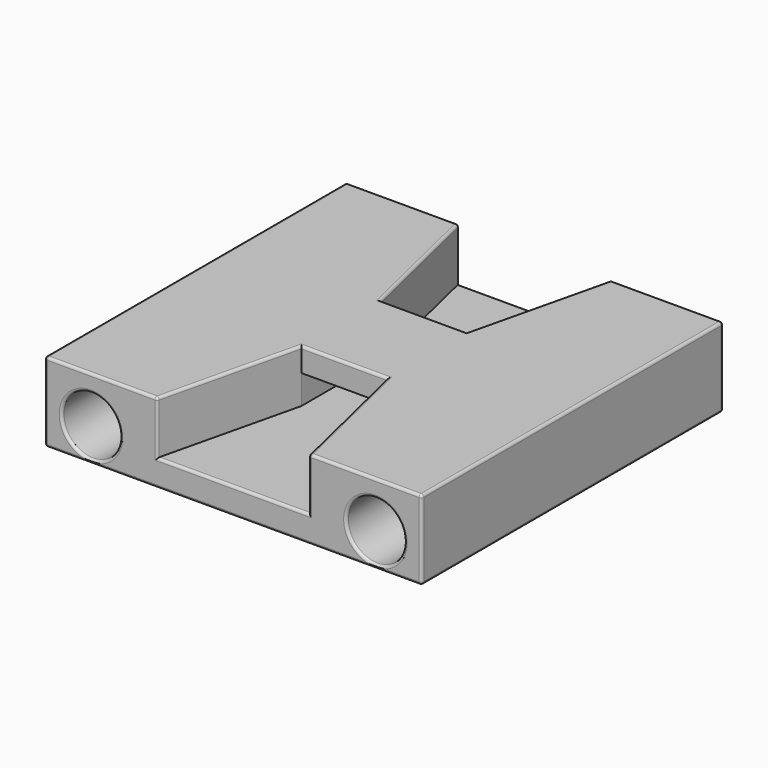
from build123d import *

# Parameters (mm, degrees)
F0_W          = 28.5
F0_H          = 28.5
F1_DEPTH      = 6
F2_W          = 6.5
F2_H          = 10.5
F3_DEPTH      = 4
F4_R          = 2.2
F5_DEPTH      = 28.501
F6_W          = 6.5
F6_H          = 2.2
F7_DEPTH      = 18.001
F8_T1_DEPTH   = 28.1
F8_T3_DEPTH   = 8.1410963279
F8_T5_DEPTH   = 8.1389034954
F8_T7_DEPTH   = 28.1
F8_T9_DEPTH   = 5.6
F8_T11_DEPTH  = 3.8
F8_S15_W      = 0.2
F8_S15_H      = 0.2
F8_T16_DEPTH  = 0.2
F8_S21_W      = 0.2
F8_S21_H      = 0.2
F8_T22_DEPTH  = 0.2
F8_T28_DEPTH  = 0.2
F8_T34_DEPTH  = 0.2
F8_S39_W      = 0.2
F8_S39_H      = 0.2
F8_T40_DEPTH  = 0.2
F8_S45_W      = 0.2
F8_S45_H      = 0.2
F8_T46_DEPTH  = 0.2
F8_T52_DEPTH  = 0.2
F8_T58_DEPTH  = 0.2
F8_S63_W      = 0.2
F8_S63_H      = 0.2
F8_T64_DEPTH  = 0.2
F8_S69_W      = 0.2
F8_S69_H      = 0.2
F8_T70_DEPTH  = 0.2
F8_S75_W      = 0.2
F8_S75_H      = 0.2
F8_T76_DEPTH  = 0.2
F8_S81_W      = 0.2
F8_S81_H      = 0.2
F8_T82_DEPTH  = 0.2
F8_T88_DEPTH  = 11.1357777684
F8_T93_DEPTH  = 7.5
F8_T99_DEPTH  = 11.13632618
F8_T104_DEPTH = 11.13632618
F8_T109_DEPTH = 7.5
F8_T115_DEPTH = 11.1357777684
F8_T120_DEPTH = 12.5041169338
F8_T130_DEPTH = 12.5041169338
F8_T141_DEPTH = 11.1357777684
F8_T145_DEPTH = 7.5
F8_T152_DEPTH = 7.5
F8_T156_DEPTH = 11.13632618
F8_T163_DEPTH = 7.5
F8_T167_DEPTH = 11.13632618
F8_T174_DEPTH = 7.5
F8_T178_DEPTH = 11.1357777684
F8_T185_DEPTH = 4.1948947572
F8_T189_DEPTH = 12.5041169338
F8_T196_DEPTH = 4.1948133503
F8_T200_DEPTH = 12.5041169338
F8_T207_DEPTH = 4.1948133503
F8_T211_DEPTH = 12.5041169338
F8_T218_DEPTH = 12.5041169338
F8_T222_DEPTH = 4.1948947572


# Not quite as in the source:
# - a fillet or chamfer that OpenCascade refuses, or shapes differently, is made with other operations: its cross-section is extruded or revolved along the edge and cut away or added


with BuildPart() as f1:
    # F0 (on Top) → F1 (new body)
    with BuildSketch(Plane.XY):
        Rectangle(F0_W, F0_H)
    extrude(amount=F1_DEPTH)

    # F2 (on face) → F3 (cut)
    with BuildSketch(Plane.XY.offset(6)):
        with Locations((0, 9)):
            Rectangle(F2_W, F2_H)
        Polygon((3.25, 14.25), (3.25, 3.75), (5.7531711645, 14.25), align=None)
        Polygon((-5.7509457693, 14.25), (-3.25, 3.75), (-3.25, 14.25), align=None)
        Polygon((-5.7509457693, -14.25), (-3.25, -14.25), (-3.25, -3.75), align=None)
        with Locations((0, -9)):
            Rectangle(F2_W, F2_H)
        Polygon((3.25, -3.75), (3.25, -14.25), (5.7531711645, -14.25), align=None)
    extrude(amount=-F3_DEPTH, mode=Mode.SUBTRACT)

    # F4 (on face) → F5 (cut, through all)
    with BuildSketch(Plane.XZ.offset(14.25)):
        with Locations((-10.75, 2.5)):
            Circle(F4_R)
        with Locations((10.75, 2.5)):
            Circle(F4_R)
    extrude(amount=-F5_DEPTH, mode=Mode.SUBTRACT)

    # F6 (on face) → F7 (cut, through all)
    with BuildSketch(Plane.XZ.offset(3.75)):
        with Locations((0, 3.1)):
            Rectangle(F6_W, F6_H)
    extrude(amount=-F7_DEPTH, mode=Mode.SUBTRACT)

    # F8: fillet of radius 0.2 on 30 edges, made by hand

    # F8_s2 → F8_t1 (cut)
    with BuildSketch(Plane.XZ.offset(-14.05)):
        with BuildLine():
            ThreePointArc((-14.05, 6), (-14.1914213562, 5.9414213562), (-14.25, 5.8))
            Line((-14.25, 5.8), (-14.25, 6))
            Line((-14.25, 6), (-14.05, 6))
        make_face()
        with BuildLine():
            ThreePointArc((14.05, 6), (14.1914213562, 5.9414213562), (14.25, 5.8))
            Line((14.25, 5.8), (14.25, 6))
            Line((14.25, 6), (14.05, 6))
        make_face()
        with BuildLine():
            ThreePointArc((14.25, 0.2), (14.1914213562, 0.0585786438), (14.05, 0))
            Line((14.05, 0), (14.25, 0))
            Line((14.25, 0), (14.25, 0.2))
        make_face()
        with BuildLine():
            ThreePointArc((-14.25, 0.2), (-14.1914213562, 0.0585786438), (-14.05, 0))
            Line((-14.05, 0), (-14.25, 0))
            Line((-14.25, 0), (-14.25, 0.2))
        make_face()
    extrude(amount=F8_T1_DEPTH, mode=Mode.SUBTRACT)

    # F8_s4 → F8_t3 (cut)
    with BuildSketch(Plane.YZ.offset(-14.05)):
        with BuildLine():
            ThreePointArc((14.25, 5.8), (14.1914213562, 5.9414213562), (14.05, 6))
            Line((14.05, 6), (14.25, 6))
            Line((14.25, 6), (14.25, 5.8))
        make_face()
        with BuildLine():
            ThreePointArc((-14.25, 5.8), (-14.1914213562, 5.9414213562), (-14.05, 6))
            Line((-14.05, 6), (-14.25, 6))
            Line((-14.25, 6), (-14.25, 5.8))
        make_face()
    extrude(amount=F8_T3_DEPTH, mode=Mode.SUBTRACT)

    # F8_s6 → F8_t5 (cut)
    with BuildSketch(Plane.YZ.offset(5.9110965046)):
        with BuildLine():
            ThreePointArc((14.25, 5.8), (14.1914213562, 5.9414213562), (14.05, 6))
            Line((14.05, 6), (14.25, 6))
            Line((14.25, 6), (14.25, 5.8))
        make_face()
        with BuildLine():
            ThreePointArc((-14.25, 5.8), (-14.1914213562, 5.9414213562), (-14.05, 6))
            Line((-14.05, 6), (-14.25, 6))
            Line((-14.25, 6), (-14.25, 5.8))
        make_face()
    extrude(amount=F8_T5_DEPTH, mode=Mode.SUBTRACT)

    # F8_s8 → F8_t7 (cut)
    with BuildSketch(Plane.YZ.offset(-14.05)):
        with BuildLine():
            ThreePointArc((-14.25, 0.2), (-14.1914213562, 0.0585786438), (-14.05, 0))
            Line((-14.05, 0), (-14.25, 0))
            Line((-14.25, 0), (-14.25, 0.2))
        make_face()
        with BuildLine():
            ThreePointArc((14.25, 0.2), (14.1914213562, 0.0585786438), (14.05, 0))
            Line((14.05, 0), (14.25, 0))
            Line((14.25, 0), (14.25, 0.2))
        make_face()
    extrude(amount=F8_T7_DEPTH, mode=Mode.SUBTRACT)

    # F8_s10 → F8_t9 (cut)
    with BuildSketch(Plane.XY.offset(0.2)):
        with BuildLine():
            ThreePointArc((-14.05, -14.25), (-14.1914213562, -14.1914213562), (-14.25, -14.05))
            Line((-14.25, -14.05), (-14.25, -14.25))
            Line((-14.25, -14.25), (-14.05, -14.25))
        make_face()
        with BuildLine():
            ThreePointArc((14.05, -14.25), (14.1914213562, -14.1914213562), (14.25, -14.05))
            Line((14.25, -14.05), (14.25, -14.25))
            Line((14.25, -14.25), (14.05, -14.25))
        make_face()
        with BuildLine():
            ThreePointArc((14.05, 14.25), (14.1914213562, 14.1914213562), (14.25, 14.05))
            Line((14.25, 14.05), (14.25, 14.25))
            Line((14.25, 14.25), (14.05, 14.25))
        make_face()
        with BuildLine():
            ThreePointArc((-14.05, 14.25), (-14.1914213562, 14.1914213562), (-14.25, 14.05))
            Line((-14.25, 14.05), (-14.25, 14.25))
            Line((-14.25, 14.25), (-14.05, 14.25))
        make_face()
    extrude(amount=F8_T9_DEPTH, mode=Mode.SUBTRACT)

    # F8_s12 → F8_t11 (cut)
    with BuildSketch(Plane.XY.offset(2)):
        with BuildLine():
            ThreePointArc((-5.9089036721, -14.25), (-5.7849442794, -14.2069524417), (-5.7143463785, -14.0963406896))
            Line((-5.7143463785, -14.0963406896), (-5.7509457693, -14.25))
            Line((-5.7509457693, -14.25), (-5.9089036721, -14.25))
        make_face()
        with BuildLine():
            ThreePointArc((5.9110965046, -14.25), (5.7871528513, -14.2069648712), (5.7165485088, -14.0963797079))
            Line((5.7165485088, -14.0963797079), (5.7531711645, -14.25))
            Line((5.7531711645, -14.25), (5.9110965046, -14.25))
        make_face()
        with BuildLine():
            ThreePointArc((5.9110965046, 14.25), (5.7871528513, 14.2069648712), (5.7165485088, 14.0963797079))
            Line((5.7165485088, 14.0963797079), (5.7531711645, 14.25))
            Line((5.7531711645, 14.25), (5.9110965046, 14.25))
        make_face()
        with BuildLine():
            ThreePointArc((-5.9089036721, 14.25), (-5.7849442794, 14.2069524417), (-5.7143463785, 14.0963406896))
            Line((-5.7143463785, 14.0963406896), (-5.7509457693, 14.25))
            Line((-5.7509457693, 14.25), (-5.9089036721, 14.25))
        make_face()
    extrude(amount=F8_T11_DEPTH, mode=Mode.SUBTRACT)


with BuildPart() as f8_tool14:
    # F8_s15 → F8_t16 (new body)
    with BuildSketch(Plane.YZ.offset(-14.05)):
        with Locations((14.15, 5.9)):
            Rectangle(F8_S15_W, F8_S15_H)
    extrude(amount=-F8_T16_DEPTH)

    # F8_s17 → F8_t18 (revolve, cut)
    with BuildSketch(Plane(origin=(-14.05, 14.05, 5.8), x_dir=(0, -0.7071067812, -0.7071067812), z_dir=(0, 0.7071067812, -0.7071067812))):
        with BuildLine():
            ThreePointArc((0, -0.2), (0.2, 0), (0, 0.2))
            Line((0, 0.2), (0, -0.2))
        make_face()
    revolve(axis=Axis((-14.05, 14.05, 5.8), (-1, 0, 0)), mode=Mode.SUBTRACT)


with BuildPart() as f1_1:
    add(f1.part)

    # F8_t13: cut F8_tool14
    add(f8_tool14.part, mode=Mode.SUBTRACT)


with BuildPart() as f8_tool20:
    # F8_s21 → F8_t22 (new body)
    with BuildSketch(Plane.YZ.offset(-14.05)):
        with Locations((-14.15, 5.9)):
            Rectangle(F8_S21_W, F8_S21_H)
    extrude(amount=-F8_T22_DEPTH)

    # F8_s23 → F8_t24 (revolve, cut)
    with BuildSketch(Plane(origin=(-14.05, -14.05, 5.8), x_dir=(0, 0.7071067812, -0.7071067812), z_dir=(0, 0.7071067812, 0.7071067812))):
        with BuildLine():
            ThreePointArc((0, -0.2), (0.2, 0), (0, 0.2))
            Line((0, 0.2), (0, -0.2))
        make_face()
    revolve(axis=Axis((-14.05, -14.05, 5.8), (-1, 0, 0)), mode=Mode.SUBTRACT)


with BuildPart() as f1_2:
    add(f1_1.part)

    # F8_t19: cut F8_tool20
    add(f8_tool20.part, mode=Mode.SUBTRACT)


with BuildPart() as f8_tool26:
    # F8_s27 → F8_t28 (new body)
    with BuildSketch(Plane.XY.offset(5.8)):
        Polygon((-5.9089036721, 14.05), (-5.9089036721, 14.25), (-5.7509457693, 14.25), (-5.7143463785, 14.0963406896), align=None)
    extrude(amount=F8_T28_DEPTH)

    # F8_s29 → F8_t30 (revolve, cut)
    with BuildSketch(Plane(origin=(-5.9089036721, 14.05, 5.8), x_dir=(-0.6197969636, -0.7847622085, 0), z_dir=(-0.7847622085, 0.6197969636, 0))):
        with BuildLine():
            ThreePointArc((0, -0.2), (0.2, 0), (0, 0.2))
            Line((0, 0.2), (0, -0.2))
        make_face()
    revolve(axis=Axis((-5.9089036721, 14.05, 5.8), (0, 0, 1)), mode=Mode.SUBTRACT)


with BuildPart() as f1_3:
    add(f1_2.part)

    # F8_t25: cut F8_tool26
    add(f8_tool26.part, mode=Mode.SUBTRACT)


with BuildPart() as f8_tool32:
    # F8_s33 → F8_t34 (new body)
    with BuildSketch(Plane.XY.offset(5.8)):
        Polygon((5.9110965046, 14.05), (5.7165485088, 14.0963797079), (5.7531711645, 14.25), (5.9110965046, 14.25), align=None)
    extrude(amount=F8_T34_DEPTH)

    # F8_s35 → F8_t36 (revolve, cut)
    with BuildSketch(Plane(origin=(5.9110965046, 14.05, 5.8), x_dir=(0.6197182668, -0.784824356, 0), z_dir=(-0.784824356, -0.6197182668, 0))):
        with BuildLine():
            ThreePointArc((0, -0.2), (0.2, 0), (0, 0.2))
            Line((0, 0.2), (0, -0.2))
        make_face()
    revolve(axis=Axis((5.9110965046, 14.05, 5.8), (0, 0, 1)), mode=Mode.SUBTRACT)


with BuildPart() as f1_4:
    add(f1_3.part)

    # F8_t31: cut F8_tool32
    add(f8_tool32.part, mode=Mode.SUBTRACT)


with BuildPart() as f8_tool38:
    # F8_s39 → F8_t40 (new body)
    with BuildSketch(Plane.XZ.offset(-14.05)):
        with Locations((14.15, 5.9)):
            Rectangle(F8_S39_W, F8_S39_H)
    extrude(amount=-F8_T40_DEPTH)

    # F8_s41 → F8_t42 (revolve, cut)
    with BuildSketch(Plane(origin=(14.05, 14.05, 5.8), x_dir=(-0.7071067812, 0, -0.7071067812), z_dir=(0.7071067812, 0, -0.7071067812))):
        with BuildLine():
            ThreePointArc((0, -0.2), (0.2, 0), (0, 0.2))
            Line((0, 0.2), (0, -0.2))
        make_face()
    revolve(axis=Axis((14.05, 14.05, 5.8), (0, 1, 0)), mode=Mode.SUBTRACT)


with BuildPart() as f1_5:
    add(f1_4.part)

    # F8_t37: cut F8_tool38
    add(f8_tool38.part, mode=Mode.SUBTRACT)


with BuildPart() as f8_tool44:
    # F8_s45 → F8_t46 (new body)
    with BuildSketch(Plane.XZ.offset(14.05)):
        with Locations((14.15, 5.9)):
            Rectangle(F8_S45_W, F8_S45_H)
    extrude(amount=F8_T46_DEPTH)

    # F8_s47 → F8_t48 (revolve, cut)
    with BuildSketch(Plane(origin=(14.05, -14.05, 5.8), x_dir=(-0.7071067812, 0, -0.7071067812), z_dir=(-0.7071067812, 0, 0.7071067812))):
        with BuildLine():
            ThreePointArc((0, -0.2), (0.2, 0), (0, 0.2))
            Line((0, 0.2), (0, -0.2))
        make_face()
    revolve(axis=Axis((14.05, -14.05, 5.8), (0, -1, 0)), mode=Mode.SUBTRACT)


with BuildPart() as f1_6:
    add(f1_5.part)

    # F8_t43: cut F8_tool44
    add(f8_tool44.part, mode=Mode.SUBTRACT)


with BuildPart() as f8_tool50:
    # F8_s51 → F8_t52 (new body)
    with BuildSketch(Plane.XY.offset(5.8)):
        Polygon((5.9110965046, -14.05), (5.9110965046, -14.25), (5.7531711645, -14.25), (5.7165485088, -14.0963797079), align=None)
    extrude(amount=F8_T52_DEPTH)

    # F8_s53 → F8_t54 (revolve, cut)
    with BuildSketch(Plane(origin=(5.9110965046, -14.05, 5.8), x_dir=(0.6197182668, 0.784824356, 0), z_dir=(0.784824356, -0.6197182668, 0))):
        with BuildLine():
            ThreePointArc((0, -0.2), (0.2, 0), (0, 0.2))
            Line((0, 0.2), (0, -0.2))
        make_face()
    revolve(axis=Axis((5.9110965046, -14.05, 5.8), (0, 0, 1)), mode=Mode.SUBTRACT)


with BuildPart() as f1_7:
    add(f1_6.part)

    # F8_t49: cut F8_tool50
    add(f8_tool50.part, mode=Mode.SUBTRACT)


with BuildPart() as f8_tool56:
    # F8_s57 → F8_t58 (new body)
    with BuildSketch(Plane.XY.offset(5.8)):
        Polygon((-5.9089036721, -14.05), (-5.9089036721, -14.25), (-5.7509457693, -14.25), (-5.7143463785, -14.0963406896), align=None)
    extrude(amount=F8_T58_DEPTH)

    # F8_s59 → F8_t60 (revolve, cut)
    with BuildSketch(Plane(origin=(-5.9089036721, -14.05, 5.8), x_dir=(-0.6197969636, 0.7847622085, 0), z_dir=(0.7847622085, 0.6197969636, 0))):
        with BuildLine():
            ThreePointArc((0, -0.2), (0.2, 0), (0, 0.2))
            Line((0, 0.2), (0, -0.2))
        make_face()
    revolve(axis=Axis((-5.9089036721, -14.05, 5.8), (0, 0, 1)), mode=Mode.SUBTRACT)


with BuildPart() as f1_8:
    add(f1_7.part)

    # F8_t55: cut F8_tool56
    add(f8_tool56.part, mode=Mode.SUBTRACT)


with BuildPart() as f8_tool62:
    # F8_s63 → F8_t64 (new body)
    with BuildSketch(Plane.XZ.offset(14.05)):
        with Locations((-14.15, 0.1)):
            Rectangle(F8_S63_W, F8_S63_H)
    extrude(amount=F8_T64_DEPTH)

    # F8_s65 → F8_t66 (revolve, cut)
    with BuildSketch(Plane(origin=(-14.05, -14.05, 0.2), x_dir=(0.7071067812, 0, 0.7071067812), z_dir=(0.7071067812, 0, -0.7071067812))):
        with BuildLine():
            ThreePointArc((0, -0.2), (0.2, 0), (0, 0.2))
            Line((0, 0.2), (0, -0.2))
        make_face()
    revolve(axis=Axis((-14.05, -14.05, 0.2), (0, -1, 0)), mode=Mode.SUBTRACT)


with BuildPart() as f1_9:
    add(f1_8.part)

    # F8_t61: cut F8_tool62
    add(f8_tool62.part, mode=Mode.SUBTRACT)


with BuildPart() as f8_tool68:
    # F8_s69 → F8_t70 (new body)
    with BuildSketch(Plane.XZ.offset(14.05)):
        with Locations((14.15, 0.1)):
            Rectangle(F8_S69_W, F8_S69_H)
    extrude(amount=F8_T70_DEPTH)

    # F8_s71 → F8_t72 (revolve, cut)
    with BuildSketch(Plane(origin=(14.05, -14.05, 0.2), x_dir=(-0.7071067812, 0, 0.7071067812), z_dir=(0.7071067812, 0, 0.7071067812))):
        with BuildLine():
            ThreePointArc((0, -0.2), (0.2, 0), (0, 0.2))
            Line((0, 0.2), (0, -0.2))
        make_face()
    revolve(axis=Axis((14.05, -14.05, 0.2), (0, -1, 0)), mode=Mode.SUBTRACT)


with BuildPart() as f1_10:
    add(f1_9.part)

    # F8_t67: cut F8_tool68
    add(f8_tool68.part, mode=Mode.SUBTRACT)


with BuildPart() as f8_tool74:
    # F8_s75 → F8_t76 (new body)
    with BuildSketch(Plane.XY.offset(0.2)):
        with Locations((14.15, 14.15)):
            Rectangle(F8_S75_W, F8_S75_H)
    extrude(amount=-F8_T76_DEPTH)

    # F8_s77 → F8_t78 (revolve, cut)
    with BuildSketch(Plane(origin=(14.05, 14.05, 0.2), x_dir=(-0.7071067812, -0.7071067812, 0), z_dir=(0.7071067812, -0.7071067812, 0))):
        with BuildLine():
            ThreePointArc((0, -0.2), (0.2, 0), (0, 0.2))
            Line((0, 0.2), (0, -0.2))
        make_face()
    revolve(axis=Axis((14.05, 14.05, 0.2), (0, 0, -1)), mode=Mode.SUBTRACT)


with BuildPart() as f1_11:
    add(f1_10.part)

    # F8_t73: cut F8_tool74
    add(f8_tool74.part, mode=Mode.SUBTRACT)


with BuildPart() as f8_tool80:
    # F8_s81 → F8_t82 (new body)
    with BuildSketch(Plane.YZ.offset(-14.05)):
        with Locations((14.15, 0.1)):
            Rectangle(F8_S81_W, F8_S81_H)
    extrude(amount=-F8_T82_DEPTH)

    # F8_s83 → F8_t84 (revolve, cut)
    with BuildSketch(Plane(origin=(-14.05, 14.05, 0.2), x_dir=(0, -0.7071067812, 0.7071067812), z_dir=(0, -0.7071067812, -0.7071067812))):
        with BuildLine():
            ThreePointArc((0, -0.2), (0.2, 0), (0, 0.2))
            Line((0, 0.2), (0, -0.2))
        make_face()
    revolve(axis=Axis((-14.05, 14.05, 0.2), (-1, 0, 0)), mode=Mode.SUBTRACT)


with BuildPart() as f1_12:
    add(f1_11.part)

    # F8_t79: cut F8_tool80
    add(f8_tool80.part, mode=Mode.SUBTRACT)


with BuildPart() as f8_tool86:
    # F8_s87 → F8_t88 (new body)
    with BuildSketch(Plane(origin=(-3.4840698832, 14.627559791, 0), x_dir=(0, 0, 1), z_dir=(0.2317034478, -0.972786468, 0))):
        with BuildLine():
            ThreePointArc((5.8, 2.2926680918), (5.9414213562, 2.3512467356), (6, 2.4926680918))
            Line((6, 2.4926680918), (6, 2.2926680918))
            Line((6, 2.2926680918), (5.8, 2.2926680918))
        make_face()
    extrude(amount=F8_T88_DEPTH)

    split(bisect_by=Plane.XZ.offset(-3.75), keep=Keep.BOTTOM)


with BuildPart() as f1_13:
    add(f1_12.part)

    # F8_t85: cut F8_tool86
    add(f8_tool86.part, mode=Mode.SUBTRACT)


with BuildPart() as f8_tool91:
    # F8_s92 → F8_t93 (new body)
    with BuildSketch(Plane.YZ.offset(-3.75)):
        with BuildLine():
            ThreePointArc((3.75, 5.8), (3.6914213562, 5.9414213562), (3.55, 6))
            Line((3.55, 6), (3.75, 6))
            Line((3.75, 6), (3.75, 5.8))
        make_face()
    extrude(amount=F8_T93_DEPTH)

    split(bisect_by=Plane(origin=(-2.2302764953, -0.5312191015, 0), x_dir=(0, 0, 1), z_dir=(0.972786468, 0.2317034478, 0)), keep=Keep.TOP)

    split(bisect_by=Plane(origin=(2.2293112911, -0.5314616896, 0), x_dir=(0, 0, 1), z_dir=(-0.9727399793, 0.2318985397, 0)), keep=Keep.TOP)


with BuildPart() as f1_14:
    add(f1_13.part)

    # F8_t90: cut F8_tool91
    add(f8_tool91.part, mode=Mode.SUBTRACT)


with BuildPart() as f8_tool97:
    # F8_s98 → F8_t99 (new body)
    with BuildSketch(Plane(origin=(0.9047394391, 3.7950916999, 0), x_dir=(0, 0, 1), z_dir=(0.2318985397, 0.9727399793, 0))):
        with BuildLine():
            ThreePointArc((5.8, 2.2917854088), (5.9414213562, 2.3503640526), (6, 2.4917854088))
            Line((6, 2.4917854088), (6, 2.2917854088))
            Line((6, 2.2917854088), (5.8, 2.2917854088))
        make_face()
    extrude(amount=F8_T99_DEPTH)

    split(bisect_by=Plane.XZ.offset(-3.75), keep=Keep.BOTTOM)


with BuildPart() as f1_15:
    add(f1_14.part)

    # F8_t96: cut F8_tool97
    add(f8_tool97.part, mode=Mode.SUBTRACT)


with BuildPart() as f8_tool102:
    # F8_s103 → F8_t104 (new body)
    with BuildSketch(Plane(origin=(3.4872372177, -14.6278413975, 0), x_dir=(0, 0, 1), z_dir=(-0.2318985397, 0.9727399793, 0))):
        with BuildLine():
            ThreePointArc((5.8, 2.2917854088), (5.9414213562, 2.3503640526), (6, 2.4917854088))
            Line((6, 2.4917854088), (6, 2.2917854088))
            Line((6, 2.2917854088), (5.8, 2.2917854088))
        make_face()
    extrude(amount=F8_T104_DEPTH)

    split(bisect_by=Plane.XZ.offset(3.75), keep=Keep.TOP)


with BuildPart() as f1_16:
    add(f1_15.part)

    # F8_t101: cut F8_tool102
    add(f8_tool102.part, mode=Mode.SUBTRACT)


with BuildPart() as f8_tool107:
    # F8_s108 → F8_t109 (new body)
    with BuildSketch(Plane.YZ.offset(3.75)):
        with BuildLine():
            ThreePointArc((-3.75, 5.8), (-3.6914213562, 5.9414213562), (-3.55, 6))
            Line((-3.55, 6), (-3.75, 6))
            Line((-3.75, 6), (-3.75, 5.8))
        make_face()
    extrude(amount=-F8_T109_DEPTH)

    split(bisect_by=Plane(origin=(-2.2302764953, 0.5312191015, 0), x_dir=(0, 0, 1), z_dir=(0.972786468, -0.2317034478, 0)), keep=Keep.TOP)

    split(bisect_by=Plane(origin=(2.2293112911, 0.5314616896, 0), x_dir=(0, 0, 1), z_dir=(-0.9727399793, -0.2318985397, 0)), keep=Keep.TOP)


with BuildPart() as f1_17:
    add(f1_16.part)

    # F8_t106: cut F8_tool107
    add(f8_tool107.part, mode=Mode.SUBTRACT)


with BuildPart() as f8_tool113:
    # F8_s114 → F8_t115 (new body)
    with BuildSketch(Plane(origin=(-0.9038717808, -3.7948258675, 0), x_dir=(0, 0, 1), z_dir=(-0.2317034478, -0.972786468, 0))):
        with BuildLine():
            ThreePointArc((5.8, 2.2926680918), (5.9414213562, 2.3512467356), (6, 2.4926680918))
            Line((6, 2.4926680918), (6, 2.2926680918))
            Line((6, 2.2926680918), (5.8, 2.2926680918))
        make_face()
    extrude(amount=F8_T115_DEPTH)

    split(bisect_by=Plane.XZ.offset(3.75), keep=Keep.TOP)


with BuildPart() as f1_18:
    add(f1_17.part)

    # F8_t112: cut F8_tool113
    add(f8_tool113.part, mode=Mode.SUBTRACT)


with BuildPart() as f8_tool118:
    # F8_s119 → F8_t120 (new body)
    with BuildSketch(Plane.YZ.offset(-6.2509457693)):
        with BuildLine():
            ThreePointArc((-14.25, 1.8), (-14.1914213562, 1.9414213562), (-14.05, 2))
            Line((-14.05, 2), (-14.25, 2))
            Line((-14.25, 2), (-14.25, 1.8))
        make_face()
    extrude(amount=F8_T120_DEPTH)

    split(bisect_by=Plane(origin=(2.2293112911, 0.5314616896, 0), x_dir=(0, 0, 1), z_dir=(-0.9727399793, -0.2318985397, 0)), keep=Keep.TOP)

    split(bisect_by=Plane(origin=(-2.2302764953, 0.5312191015, 0), x_dir=(0, 0, 1), z_dir=(0.972786468, -0.2317034478, 0)), keep=Keep.TOP)


with BuildPart() as f1_19:
    add(f1_18.part)

    # F8_t117: cut F8_tool118
    add(f8_tool118.part, mode=Mode.SUBTRACT)

    # F8_s123 → F8_t124 (revolve, cut)
    with BuildSketch(Plane.XY.offset(2.5)):
        with BuildLine():
            ThreePointArc((-8.35, -14.25), (-8.4914213562, -14.1914213562), (-8.55, -14.05))
            Line((-8.55, -14.05), (-8.55, -14.25))
            Line((-8.55, -14.25), (-8.35, -14.25))
        make_face()
    revolve(axis=Axis((-10.75, -14.25, 2.5), (0, -1, 0)), mode=Mode.SUBTRACT)

    # F8_s125 → F8_t126 (revolve, cut)
    with BuildSketch(Plane.XY.offset(2.5)):
        with BuildLine():
            ThreePointArc((13.15, -14.25), (13.0085786438, -14.1914213562), (12.95, -14.05))
            Line((12.95, -14.05), (12.95, -14.25))
            Line((12.95, -14.25), (13.15, -14.25))
        make_face()
    revolve(axis=Axis((10.75, -14.25, 2.5), (0, -1, 0)), mode=Mode.SUBTRACT)


with BuildPart() as f8_tool128:
    # F8_s129 → F8_t130 (new body)
    with BuildSketch(Plane.YZ.offset(6.2531711645)):
        with BuildLine():
            ThreePointArc((14.25, 1.8), (14.1914213562, 1.9414213562), (14.05, 2))
            Line((14.05, 2), (14.25, 2))
            Line((14.25, 2), (14.25, 1.8))
        make_face()
    extrude(amount=-F8_T130_DEPTH)

    split(bisect_by=Plane(origin=(-2.2302764953, -0.5312191015, 0), x_dir=(0, 0, 1), z_dir=(0.972786468, 0.2317034478, 0)), keep=Keep.TOP)

    split(bisect_by=Plane(origin=(2.2293112911, -0.5314616896, 0), x_dir=(0, 0, 1), z_dir=(-0.9727399793, 0.2318985397, 0)), keep=Keep.TOP)


with BuildPart() as f1_20:
    add(f1_19.part)

    # F8_t127: cut F8_tool128
    add(f8_tool128.part, mode=Mode.SUBTRACT)

    # F8_s133 → F8_t134 (revolve, cut)
    with BuildSketch(Plane.XY.offset(2.5)):
        with BuildLine():
            ThreePointArc((12.95, 14.05), (13.0085786438, 14.1914213562), (13.15, 14.25))
            Line((13.15, 14.25), (12.95, 14.25))
            Line((12.95, 14.25), (12.95, 14.05))
        make_face()
    revolve(axis=Axis((10.75, 14.25, 2.5), (0, -1, 0)), mode=Mode.SUBTRACT)

    # F8_s135 → F8_t136 (revolve, cut)
    with BuildSketch(Plane.XY.offset(2.5)):
        with BuildLine():
            ThreePointArc((-8.35, 14.25), (-8.4914213562, 14.1914213562), (-8.55, 14.05))
            Line((-8.55, 14.05), (-8.55, 14.25))
            Line((-8.55, 14.25), (-8.35, 14.25))
        make_face()
    revolve(axis=Axis((-10.75, 14.25, 2.5), (0, -1, 0)), mode=Mode.SUBTRACT)


with BuildPart() as f8_tool139:
    # F8_s140 → F8_t141 (new body)
    with BuildSketch(Plane(origin=(-3.4840698832, 14.627559791, 0), x_dir=(0, 0, 1), z_dir=(0.2317034478, -0.972786468, 0))):
        with BuildLine():
            ThreePointArc((5.8, 2.2926680918), (5.9414213562, 2.3512467356), (6, 2.4926680918))
            Line((6, 2.4926680918), (6, 2.2926680918))
            Line((6, 2.2926680918), (5.8, 2.2926680918))
        make_face()
    extrude(amount=F8_T141_DEPTH)

    split(bisect_by=Plane.XZ.offset(-3.75), keep=Keep.TOP)


with BuildPart() as f8_tool143:
    # F8_s144 → F8_t145 (new body)
    with BuildSketch(Plane.YZ.offset(-3.75)):
        with BuildLine():
            ThreePointArc((3.75, 5.8), (3.6914213562, 5.9414213562), (3.55, 6))
            Line((3.55, 6), (3.75, 6))
            Line((3.75, 6), (3.75, 5.8))
        make_face()
    extrude(amount=F8_T145_DEPTH)

    split(bisect_by=Plane(origin=(-2.2302764953, -0.5312191015, 0), x_dir=(0, 0, 1), z_dir=(-0.972786468, -0.2317034478, 0)), keep=Keep.TOP)


with BuildPart() as f8_tool139_1:
    add(f8_tool139.part)

    # F8_t147: intersect F8_tool143
    add(f8_tool143.part, mode=Mode.INTERSECT)


with BuildPart() as f1_21:
    add(f1_20.part)

    # F8_t137: cut F8_tool139
    add(f8_tool139_1.part, mode=Mode.SUBTRACT)


with BuildPart() as f8_tool150:
    # F8_s151 → F8_t152 (new body)
    with BuildSketch(Plane.YZ.offset(-3.75)):
        with BuildLine():
            ThreePointArc((3.75, 5.8), (3.6914213562, 5.9414213562), (3.55, 6))
            Line((3.55, 6), (3.75, 6))
            Line((3.75, 6), (3.75, 5.8))
        make_face()
    extrude(amount=F8_T152_DEPTH)

    split(bisect_by=Plane(origin=(2.2293112911, -0.5314616896, 0), x_dir=(0, 0, 1), z_dir=(0.9727399793, -0.2318985397, 0)), keep=Keep.TOP)


with BuildPart() as f8_tool154:
    # F8_s155 → F8_t156 (new body)
    with BuildSketch(Plane(origin=(0.9047394391, 3.7950916999, 0), x_dir=(0, 0, 1), z_dir=(0.2318985397, 0.9727399793, 0))):
        with BuildLine():
            ThreePointArc((5.8, 2.2917854088), (5.9414213562, 2.3503640526), (6, 2.4917854088))
            Line((6, 2.4917854088), (6, 2.2917854088))
            Line((6, 2.2917854088), (5.8, 2.2917854088))
        make_face()
    extrude(amount=F8_T156_DEPTH)

    split(bisect_by=Plane.XZ.offset(-3.75), keep=Keep.TOP)


with BuildPart() as f8_tool150_1:
    add(f8_tool150.part)

    # F8_t158: intersect F8_tool154
    add(f8_tool154.part, mode=Mode.INTERSECT)


with BuildPart() as f1_22:
    add(f1_21.part)

    # F8_t148: cut F8_tool150
    add(f8_tool150_1.part, mode=Mode.SUBTRACT)


with BuildPart() as f8_tool161:
    # F8_s162 → F8_t163 (new body)
    with BuildSketch(Plane.YZ.offset(3.75)):
        with BuildLine():
            ThreePointArc((-3.75, 5.8), (-3.6914213562, 5.9414213562), (-3.55, 6))
            Line((-3.55, 6), (-3.75, 6))
            Line((-3.75, 6), (-3.75, 5.8))
        make_face()
    extrude(amount=-F8_T163_DEPTH)

    split(bisect_by=Plane(origin=(2.2293112911, 0.5314616896, 0), x_dir=(0, 0, 1), z_dir=(0.9727399793, 0.2318985397, 0)), keep=Keep.TOP)


with BuildPart() as f8_tool165:
    # F8_s166 → F8_t167 (new body)
    with BuildSketch(Plane(origin=(3.4872372177, -14.6278413975, 0), x_dir=(0, 0, 1), z_dir=(-0.2318985397, 0.9727399793, 0))):
        with BuildLine():
            ThreePointArc((5.8, 2.2917854088), (5.9414213562, 2.3503640526), (6, 2.4917854088))
            Line((6, 2.4917854088), (6, 2.2917854088))
            Line((6, 2.2917854088), (5.8, 2.2917854088))
        make_face()
    extrude(amount=F8_T167_DEPTH)

    split(bisect_by=Plane.XZ.offset(3.75), keep=Keep.BOTTOM)


with BuildPart() as f8_tool161_1:
    add(f8_tool161.part)

    # F8_t169: intersect F8_tool165
    add(f8_tool165.part, mode=Mode.INTERSECT)


with BuildPart() as f1_23:
    add(f1_22.part)

    # F8_t159: cut F8_tool161
    add(f8_tool161_1.part, mode=Mode.SUBTRACT)


with BuildPart() as f8_tool172:
    # F8_s173 → F8_t174 (new body)
    with BuildSketch(Plane.YZ.offset(3.75)):
        with BuildLine():
            ThreePointArc((-3.75, 5.8), (-3.6914213562, 5.9414213562), (-3.55, 6))
            Line((-3.55, 6), (-3.75, 6))
            Line((-3.75, 6), (-3.75, 5.8))
        make_face()
    extrude(amount=-F8_T174_DEPTH)

    split(bisect_by=Plane(origin=(-2.2302764953, 0.5312191015, 0), x_dir=(0, 0, 1), z_dir=(-0.972786468, 0.2317034478, 0)), keep=Keep.TOP)


with BuildPart() as f8_tool176:
    # F8_s177 → F8_t178 (new body)
    with BuildSketch(Plane(origin=(-0.9038717808, -3.7948258675, 0), x_dir=(0, 0, 1), z_dir=(-0.2317034478, -0.972786468, 0))):
        with BuildLine():
            ThreePointArc((5.8, 2.2926680918), (5.9414213562, 2.3512467356), (6, 2.4926680918))
            Line((6, 2.4926680918), (6, 2.2926680918))
            Line((6, 2.2926680918), (5.8, 2.2926680918))
        make_face()
    extrude(amount=F8_T178_DEPTH)

    split(bisect_by=Plane.XZ.offset(3.75), keep=Keep.BOTTOM)


with BuildPart() as f8_tool172_1:
    add(f8_tool172.part)

    # F8_t180: intersect F8_tool176
    add(f8_tool176.part, mode=Mode.INTERSECT)


with BuildPart() as f1_24:
    add(f1_23.part)

    # F8_t170: cut F8_tool172
    add(f8_tool172_1.part, mode=Mode.SUBTRACT)


with BuildPart() as f8_tool183:
    # F8_s184 → F8_t185 (new body)
    with BuildSketch(Plane.XY.offset(5.8)):
        with BuildLine():
            ThreePointArc((-5.9089036721, -14.25), (-5.7849442794, -14.2069524417), (-5.7143463785, -14.0963406896))
            Line((-5.7143463785, -14.0963406896), (-5.7509457693, -14.25))
            Line((-5.7509457693, -14.25), (-5.9089036721, -14.25))
        make_face()
    extrude(amount=-F8_T185_DEPTH)

    split(bisect_by=Plane.XY.offset(2), keep=Keep.BOTTOM)


with BuildPart() as f8_tool187:
    # F8_s188 → F8_t189 (new body)
    with BuildSketch(Plane.YZ.offset(-6.2509457693)):
        with BuildLine():
            ThreePointArc((-14.25, 1.8), (-14.1914213562, 1.9414213562), (-14.05, 2))
            Line((-14.05, 2), (-14.25, 2))
            Line((-14.25, 2), (-14.25, 1.8))
        make_face()
    extrude(amount=F8_T189_DEPTH)

    split(bisect_by=Plane(origin=(-2.2302764953, 0.5312191015, 0), x_dir=(0, 0, 1), z_dir=(-0.972786468, 0.2317034478, 0)), keep=Keep.TOP)


with BuildPart() as f8_tool183_1:
    add(f8_tool183.part)

    # F8_t191: intersect F8_tool187
    add(f8_tool187.part, mode=Mode.INTERSECT)


with BuildPart() as f1_25:
    add(f1_24.part)

    # F8_t181: cut F8_tool183
    add(f8_tool183_1.part, mode=Mode.SUBTRACT)


with BuildPart() as f8_tool194:
    # F8_s195 → F8_t196 (new body)
    with BuildSketch(Plane.XY.offset(5.8)):
        with BuildLine():
            ThreePointArc((5.9110965046, -14.25), (5.7871528513, -14.2069648712), (5.7165485088, -14.0963797079))
            Line((5.7165485088, -14.0963797079), (5.7531711645, -14.25))
            Line((5.7531711645, -14.25), (5.9110965046, -14.25))
        make_face()
    extrude(amount=-F8_T196_DEPTH)

    split(bisect_by=Plane.XY.offset(2), keep=Keep.BOTTOM)


with BuildPart() as f8_tool198:
    # F8_s199 → F8_t200 (new body)
    with BuildSketch(Plane.YZ.offset(-6.2509457693)):
        with BuildLine():
            ThreePointArc((-14.25, 1.8), (-14.1914213562, 1.9414213562), (-14.05, 2))
            Line((-14.05, 2), (-14.25, 2))
            Line((-14.25, 2), (-14.25, 1.8))
        make_face()
    extrude(amount=F8_T200_DEPTH)

    split(bisect_by=Plane(origin=(2.2293112911, 0.5314616896, 0), x_dir=(0, 0, 1), z_dir=(0.9727399793, 0.2318985397, 0)), keep=Keep.TOP)


with BuildPart() as f8_tool194_1:
    add(f8_tool194.part)

    # F8_t202: intersect F8_tool198
    add(f8_tool198.part, mode=Mode.INTERSECT)


with BuildPart() as f1_26:
    add(f1_25.part)

    # F8_t192: cut F8_tool194
    add(f8_tool194_1.part, mode=Mode.SUBTRACT)


with BuildPart() as f8_tool205:
    # F8_s206 → F8_t207 (new body)
    with BuildSketch(Plane.XY.offset(5.8)):
        with BuildLine():
            ThreePointArc((5.9110965046, 14.25), (5.7871528513, 14.2069648712), (5.7165485088, 14.0963797079))
            Line((5.7165485088, 14.0963797079), (5.7531711645, 14.25))
            Line((5.7531711645, 14.25), (5.9110965046, 14.25))
        make_face()
    extrude(amount=-F8_T207_DEPTH)

    split(bisect_by=Plane.XY.offset(2), keep=Keep.BOTTOM)


with BuildPart() as f8_tool209:
    # F8_s210 → F8_t211 (new body)
    with BuildSketch(Plane.YZ.offset(6.2531711645)):
        with BuildLine():
            ThreePointArc((14.25, 1.8), (14.1914213562, 1.9414213562), (14.05, 2))
            Line((14.05, 2), (14.25, 2))
            Line((14.25, 2), (14.25, 1.8))
        make_face()
    extrude(amount=-F8_T211_DEPTH)

    split(bisect_by=Plane(origin=(2.2293112911, -0.5314616896, 0), x_dir=(0, 0, 1), z_dir=(0.9727399793, -0.2318985397, 0)), keep=Keep.TOP)


with BuildPart() as f8_tool205_1:
    add(f8_tool205.part)

    # F8_t213: intersect F8_tool209
    add(f8_tool209.part, mode=Mode.INTERSECT)


with BuildPart() as f1_27:
    add(f1_26.part)

    # F8_t203: cut F8_tool205
    add(f8_tool205_1.part, mode=Mode.SUBTRACT)


with BuildPart() as f8_tool216:
    # F8_s217 → F8_t218 (new body)
    with BuildSketch(Plane.YZ.offset(6.2531711645)):
        with BuildLine():
            ThreePointArc((14.25, 1.8), (14.1914213562, 1.9414213562), (14.05, 2))
            Line((14.05, 2), (14.25, 2))
            Line((14.25, 2), (14.25, 1.8))
        make_face()
    extrude(amount=-F8_T218_DEPTH)

    split(bisect_by=Plane(origin=(-2.2302764953, -0.5312191015, 0), x_dir=(0, 0, 1), z_dir=(-0.972786468, -0.2317034478, 0)), keep=Keep.TOP)


with BuildPart() as f8_tool220:
    # F8_s221 → F8_t222 (new body)
    with BuildSketch(Plane.XY.offset(5.8)):
        with BuildLine():
            ThreePointArc((-5.9089036721, 14.25), (-5.7849442794, 14.2069524417), (-5.7143463785, 14.0963406896))
            Line((-5.7143463785, 14.0963406896), (-5.7509457693, 14.25))
            Line((-5.7509457693, 14.25), (-5.9089036721, 14.25))
        make_face()
    extrude(amount=-F8_T222_DEPTH)

    split(bisect_by=Plane.XY.offset(2), keep=Keep.BOTTOM)


with BuildPart() as f8_tool216_1:
    add(f8_tool216.part)

    # F8_t224: intersect F8_tool220
    add(f8_tool220.part, mode=Mode.INTERSECT)


with BuildPart() as f1_28:
    add(f1_27.part)

    # F8_t214: cut F8_tool216
    add(f8_tool216_1.part, mode=Mode.SUBTRACT)


solid = f1_28.part
